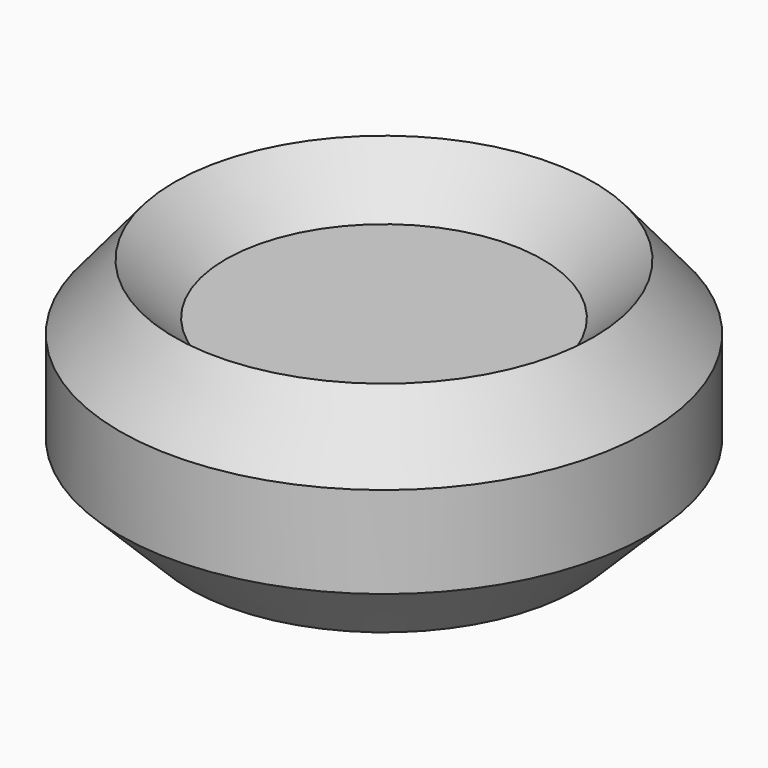
from build123d import *

# Parameters (mm, degrees)
F0_R     = 37.5
F1_DEPTH = 35
F3_R     = 22.5
F4_DEPTH = 10


# Not quite as in the source:
# - a fillet or chamfer that OpenCascade refuses, or shapes differently, is made with other operations: its cross-section is extruded or revolved along the edge and cut away or added


with BuildPart() as f1:
    # F0 (on Top) → F1 (new body)
    with BuildSketch(Plane.XY):
        Circle(F0_R)
    extrude(amount=F1_DEPTH)

    # F2: chamfer of 10 x 12 on 1 edges, made by hand

    # F2_s1 → F2_t2 (revolve, cut)
    with BuildSketch(Plane.XZ):
        Polygon((37.5, 23), (27.5, 35), (37.5, 35), align=None)
    revolve(axis=Axis((0, 0, 35), (0, 0, 1)), mode=Mode.SUBTRACT)

    # F3 (on face) → F4 (cut)
    with BuildSketch(Plane.XY.offset(35)):
        Circle(F3_R)
    extrude(amount=-F4_DEPTH, mode=Mode.SUBTRACT)

    # F5: chamfer of 10 on 2 edges, made by hand


with BuildPart() as f5_tool2:
    # F5_s3 → F5_t4 (revolve)
    with BuildSketch(Plane.XZ):
        Polygon((32.5, 35), (22.5, 25), (22.5, 35), align=None)
    revolve(axis=Axis((0, 0, 35), (0, 0, 1)))

    split(bisect_by=Plane.XY.offset(25), keep=Keep.TOP)


with BuildPart() as f1_1:
    add(f1.part)

    # F5_t1: cut F5_tool2
    add(f5_tool2.part, mode=Mode.SUBTRACT)

    # F5_s6 → F5_t7 (revolve, cut)
    with BuildSketch(Plane.XZ):
        Polygon((37.5, 10), (27.5, 0), (37.5, 0), align=None)
    revolve(axis=Axis((0, 0, 0), (0, 0, 1)), mode=Mode.SUBTRACT)


solid = f1_1.part
